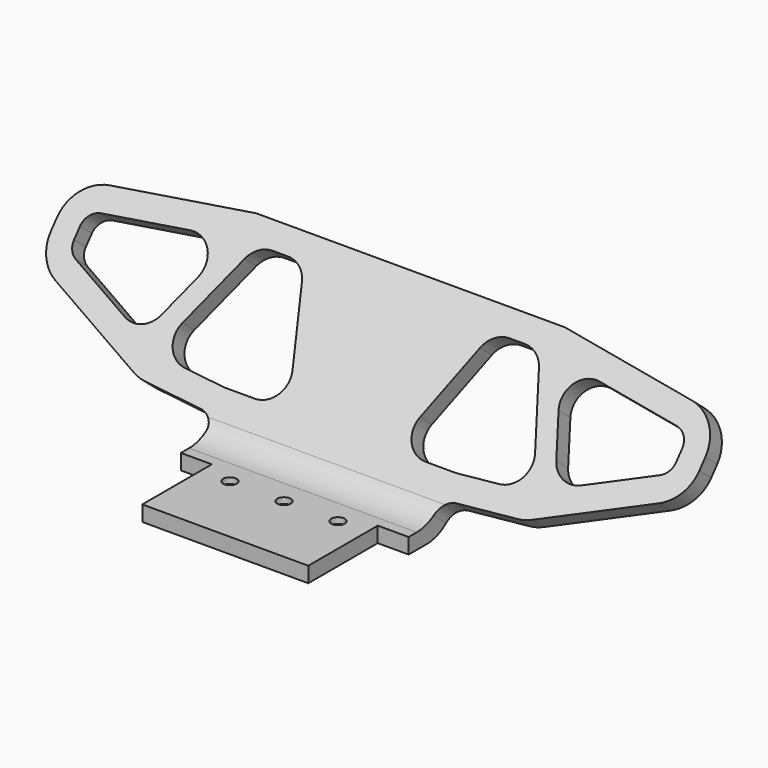
from build123d import *

# Parameters (mm, degrees)
F0_R     = 0.875
F1_DEPTH = 2
F4_DEPTH = 2.5
F6_DEPTH = 25.4913661255
F7_R     = 5
F8_R     = 3
F9_SIZE  = 1.25


with BuildPart() as f1:
    # F0 (on Top) → F1 (new body)
    with BuildSketch(Plane.XY):
        Polygon((14.75, 0), (0, 0), (-14.75, 0), (-14.75, -5.25), (-10.75, -5.25), (-10.75, -16.5), (0, -16.5), (10.75, -16.5), (10.75, -5.25), (14.75, -5.25), align=None)
        with Locations((-7, -7)):
            Circle(F0_R, mode=Mode.SUBTRACT)
        with Locations((0, -7)):
            Circle(F0_R, mode=Mode.SUBTRACT)
        with Locations((7, -7)):
            Circle(F0_R, mode=Mode.SUBTRACT)
    extrude(amount=F1_DEPTH)

    # F3 (on face) → F4 (join)
    with BuildSketch(Plane(origin=(0, 0, 0), x_dir=(-1, 0, 0), z_dir=(0, 0.7660444431, -0.6427876097))):
        with BuildLine():
            Line((-14.75, 0), (14.75, 0))
            Line((14.75, 0), (14.75, 1.3812757004))
            ThreePointArc((14.75, 1.3812757004), (15.2754453264, 2.7324561156), (16.5756885145, 3.3736650966))
            Line((16.5756885145, 3.3736650966), (24.147387942, 4.0361029601))
            ThreePointArc((24.147387942, 4.0361029601), (24.9815296917, 4.1810344722), (25.7792604037, 4.464624516))
            Line((25.7792604037, 4.464624516), (39.0676511754, 10.5))
            ThreePointArc((39.0676511754, 10.5), (41.2034661814, 12.3448936136), (42, 15.0524519346))
            Line((42, 15.0524519346), (42, 16.5491437132))
            ThreePointArc((42, 16.5491437132), (40.7746857814, 19.8281294179), (37.6993010994, 21.5))
            Line((37.6993010994, 21.5), (20, 24))
            Line((20, 24), (0, 24))
            Line((0, 24), (-20, 24))
            Line((-20, 24), (-37.6993010994, 21.5))
            ThreePointArc((-37.6993010994, 21.5), (-40.7746857814, 19.8281294179), (-42, 16.5491437132))
            Line((-42, 16.5491437132), (-42, 15.0524519346))
            ThreePointArc((-42, 15.0524519346), (-41.2034661814, 12.3448936136), (-39.0676511754, 10.5))
            Line((-39.0676511754, 10.5), (-25.7792604037, 4.464624516))
            ThreePointArc((-25.7792604037, 4.464624516), (-24.9815296917, 4.1810344722), (-24.147387942, 4.0361029601))
            Line((-24.147387942, 4.0361029601), (-16.5756885145, 3.3736650966))
            ThreePointArc((-16.5756885145, 3.3736650966), (-15.2754453264, 2.7324561156), (-14.75, 1.3812757004))
            Line((-14.75, 1.3812757004), (-14.75, 0))
        make_face()
    extrude(amount=-F4_DEPTH)

    # F5 (on face) → F6 (cut, through all)
    with BuildSketch(Plane(origin=(0, 0, 0), x_dir=(-1, 0, 0), z_dir=(0, 0.7660444431, -0.6427876097))):
        with BuildLine():
            Line((-21.098955464, 20.8149952552), (-37.2797204398, 18.5294862279))
            ThreePointArc((-37.2797204398, 18.5294862279), (-38.5098743126, 17.8607379951), (-39, 16.5491437132))
            Line((-39, 16.5491437132), (-39, 15.0524519346))
            ThreePointArc((-39, 15.0524519346), (-38.6813864726, 13.9694286062), (-37.8270604702, 13.2314711608))
            Line((-37.8270604702, 13.2314711608), (-26.8148956657, 8.2299212644))
            Line((-26.8148956657, 8.2299212644), (-21.098955464, 20.8149952552))
        make_face()
        with BuildLine():
            Line((-12.2691561683, 21), (-18.2691561683, 21))
            Line((-18.2691561683, 21), (-24.5386696984, 7.1960956767))
            ThreePointArc((-24.5386696984, 7.1960956767), (-24.2195774136, 7.0826596592), (-23.8859207138, 7.0246870544))
            Line((-23.8859207138, 7.0246870544), (-15.0312071638, 6.25))
            Line((-15.0312071638, 6.25), (-6.732866085, 6.25))
            Line((-6.732866085, 6.25), (-12.2691561683, 21))
        make_face()
        with BuildLine():
            Line((18.2691561683, 21), (12.2691561683, 21))
            Line((12.2691561683, 21), (6.732866085, 6.25))
            Line((6.732866085, 6.25), (15.0312071638, 6.25))
            Line((15.0312071638, 6.25), (23.8859207138, 7.0246870544))
            ThreePointArc((23.8859207138, 7.0246870544), (24.2195774136, 7.0826596592), (24.5386696984, 7.1960956767))
            Line((24.5386696984, 7.1960956767), (18.2691561683, 21))
        make_face()
        with BuildLine():
            Line((37.2797204398, 18.5294862279), (21.098955464, 20.8149952552))
            Line((21.098955464, 20.8149952552), (26.8148956657, 8.2299212644))
            Line((26.8148956657, 8.2299212644), (37.8270604702, 13.2314711608))
            ThreePointArc((37.8270604702, 13.2314711608), (38.6813864726, 13.9694286062), (39, 15.0524519346))
            Line((39, 15.0524519346), (39, 16.5491437132))
            ThreePointArc((39, 16.5491437132), (38.5098743126, 17.8607379951), (37.2797204398, 18.5294862279))
        make_face()
    extrude(amount=-F6_DEPTH, mode=Mode.SUBTRACT)

    # F7 (call 1 of 2: OpenCascade refuses the feature's edges together)
    f7_edges = [f1.edges().sort_by_distance(p)[0] for p in [
        (0, -1.585319, 2),
    ]]
    fillet(f7_edges, radius=F7_R)

    # F7#2 (call 2 of 2)
    f7_2_edges = [f1.edges().sort_by_distance(p)[0] for p in [
        (0, 0, 0),
    ]]
    fillet(f7_2_edges, radius=F7_R)

    # F8
    f8_edges = [f1.edges().sort_by_distance(p)[0] for p in [
        (-21.098955, 12.422065, 16.748696),
        (-26.814896, 4.332536, 7.10797),
        (-24.53867, 3.668006, 6.316014),
        (-6.732866, 3.059867, 5.591262),
        (-12.269156, 12.540984, 16.890418),
        (-18.269156, 12.540984, 16.890418),
        (12.269156, 12.540984, 16.890418),
        (18.269156, 12.540984, 16.890418),
        (24.53867, 3.668006, 6.316014),
        (6.732866, 3.059867, 5.591262),
        (26.814896, 4.332536, 7.10797),
        (21.098955, 12.422065, 16.748696),
    ]]
    fillet(f8_edges, radius=F8_R)

    # F9
    f9_edges = [f1.edges().sort_by_distance(p)[0] for p in [
        (-7.875, -7, 0),
        (-0.875, -7, 0),
        (6.125, -7, 0),
    ]]
    chamfer(f9_edges, length=F9_SIZE)


solid = f1.part
